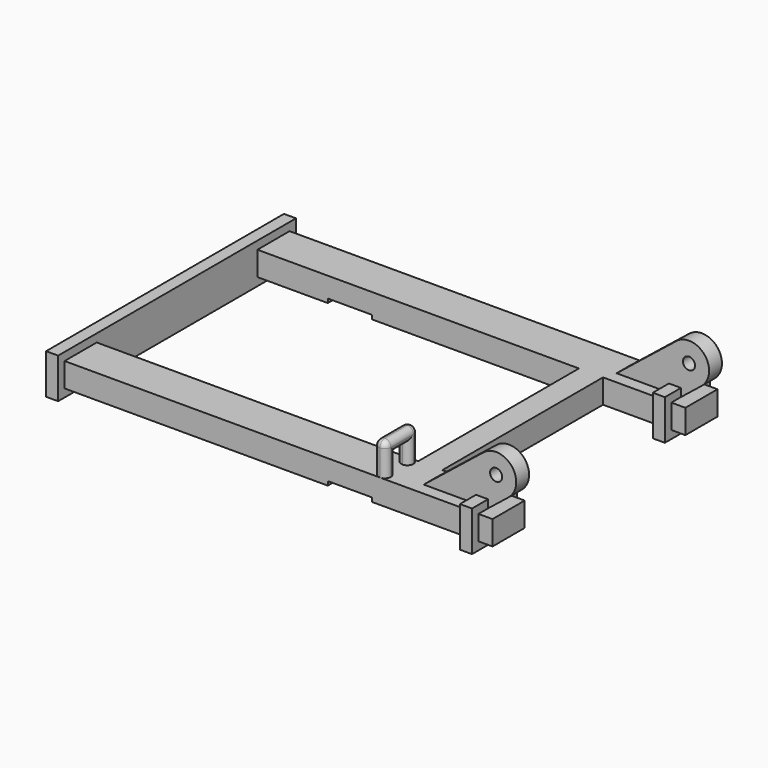
from build123d import *

# Parameters (mm, degrees)
F0_W          = 1.524
F0_H          = 12.7
F1_DEPTH      = 1.524
F2_W          = 0.762
F2_H          = 18.796
F2_H_2        = 3.556
F3_DEPTH      = 0.508
F3_DEPTH_BACK = 2.032
F4_R          = 0.381
F5_DEPTH      = 1.778
F7_DEPTH      = 0.762
F9_W          = 2.794
F9_H          = 2.54
F10_DEPTH     = 0.254
F11_W         = 2.54
F11_H         = 1.524
F12_DEPTH     = 0.889
F13_W         = 2.54
F13_H         = 1.524
F14_DEPTH     = 0.889
F15_W         = 0.762
F15_H         = 0.762
F16_DEPTH     = 2.032
F17_W         = 0.762
F17_H         = 0.762
F18_DEPTH     = 1.016
F19_R         = 0.38099


# Not quite as in the source:
# - a fillet or chamfer is up to 0.001 mm smaller than in the source, because OpenCascade refuses the exact size
# - a pattern or mirror of a feature is missing from the dataset's text; its kind, count and spacing are read off the source's solid


with BuildPart() as f1:
    # F0 (on Top) → F1 (new body)
    with BuildSketch(Plane.XY):
        Polygon((-12.7, 17.78), (-12.7, 15.24), (7.62, 15.24), (9.144, 15.24), (12.7, 15.24), (12.7, 17.78), align=None)
        Polygon((-12.7, 0), (-12.7, 2.54), (-12.7, 15.24), (-12.7, 17.78), (-12.7, 18.288), (-13.462, 18.288), (-13.462, -0.508), (-12.7, -0.508), align=None)
        Polygon((7.62, 2.54), (-12.7, 2.54), (-12.7, 0), (12.7, 0), (12.7, 2.54), (9.144, 2.54), align=None)
        with Locations((8.382, 8.89)):
            Rectangle(F0_W, F0_H)
        Polygon((12.7, 2.54), (12.7, 0), (12.7, -0.508), (13.462, -0.508), (13.462, 3.048), (12.7, 3.048), align=None)
        Polygon((12.7, 18.288), (12.7, 17.78), (12.7, 15.24), (12.7, 14.732), (13.462, 14.732), (13.462, 18.288), align=None)
    extrude(amount=F1_DEPTH)

    # F2 (on face) → F3 (join, two sides)
    with BuildSketch(Plane.XY.offset(1.524)) as f3_sk:
        with Locations((-13.081, 8.89)):
            Rectangle(F2_W, F2_H)
        with Locations((13.081, 16.51)):
            Rectangle(F2_W, F2_H_2)
        with Locations((13.081, 1.27)):
            Rectangle(F2_W, F2_H_2)
    extrude(amount=F3_DEPTH)
    extrude(f3_sk.sketch, amount=-F3_DEPTH_BACK)

    # F4 (on face) → F5 (join)
    with BuildSketch(Plane.XZ):
        with BuildLine():
            Line((13.462, 1.524), (14.762993756, 2.564001561))
            ThreePointArc((14.762993756, 2.564001561), (14.961998439, 4.348993756), (13.177006244, 4.547998439))
            Line((13.177006244, 4.547998439), (9.3941243381, 1.524))
            Line((9.3941243381, 1.524), (13.462, 1.524))
        make_face()
        with Locations((13.97, 3.556)):
            Circle(F4_R, mode=Mode.SUBTRACT)
    f5 = extrude(amount=-F5_DEPTH)

    # F5_copies: F5 across plane
    add(f5.mirror(Plane.ZX.offset(8.89)))

    # F6 (on face) → F7 (cut)
    with BuildSketch(Plane.XZ):
        with BuildLine():
            Line((13.177006244, 4.547998439), (9.3941243381, 1.524))
            Line((9.3941243381, 1.524), (12.7, 1.524))
            Line((12.7, 1.524), (12.7, 2.032))
            Line((12.7, 2.032), (13.462, 2.032))
            Line((13.462, 2.032), (13.462, 1.524))
            Line((13.462, 1.524), (14.762993756, 2.564001561))
            ThreePointArc((14.762993756, 2.564001561), (14.961998439, 4.348993756), (13.177006244, 4.547998439))
        make_face()
    f7 = extrude(amount=-F7_DEPTH, mode=Mode.SUBTRACT)

    # F7_copies: F7 across plane
    add(f7.mirror(Plane.ZX.offset(8.89)), mode=Mode.SUBTRACT)

    # F9 (on face) → F10 (cut)
    with BuildSketch(Plane(origin=(0, 0, 0), x_dir=(1, 0, 0), z_dir=(0, 0, -1))):
        with Locations((5.334, -1.27)):
            Rectangle(F9_W, F9_H)
        with Locations((-6.858, -16.51)):
            Rectangle(F9_W, F9_H)
    extrude(amount=-F10_DEPTH, mode=Mode.SUBTRACT)

    # F11 (on face) → F12 (join)
    with BuildSketch(Plane.YZ.offset(13.462)):
        with Locations((1.27, 0.762)):
            Rectangle(F11_W, F11_H)
    extrude(amount=F12_DEPTH)

    # F13 (on face) → F14 (join)
    with BuildSketch(Plane.YZ.offset(13.462)):
        with Locations((16.51, 0.762)):
            Rectangle(F13_W, F13_H)
    extrude(amount=F14_DEPTH)

    # F15 (on face) → F16 (join)
    with BuildSketch(Plane.XY.offset(1.524)):
        with Locations((7.239, 2.159)):
            Rectangle(F15_W, F15_H)
        with Locations((7.239, 0.381)):
            Rectangle(F15_W, F15_H)
    extrude(amount=F16_DEPTH)

    # F17 (on face) → F18 (join, through all)
    with BuildSketch(Plane.XZ.offset(-1.778)):
        with Locations((7.239, 3.175)):
            Rectangle(F17_W, F17_H)
    extrude(amount=F18_DEPTH)

    # F19 (radius 0.381 in the source; OpenCascade refuses exactly that, so slightly less here)
    f19_edges = [f1.edges().sort_by_distance(p)[0] for p in [
        (6.858, 2.54, 2.54),
        (7.62, 2.54, 2.54),
        (7.239, 2.54, 3.556),
        (7.62, 1.27, 3.556),
        (6.858, 1.27, 3.556),
        (6.858, 1.27, 2.794),
        (6.858, 1.778, 2.159),
        (6.858, 0.762, 2.159),
        (7.62, 0.762, 2.159),
        (6.858, 0, 2.54),
        (7.239, 0, 3.556),
        (7.62, 1.27, 2.794),
        (7.62, 0, 2.54),
        (7.62, 1.778, 2.159),
    ]]
    fillet(f19_edges, radius=F19_R)


solid = f1.part
